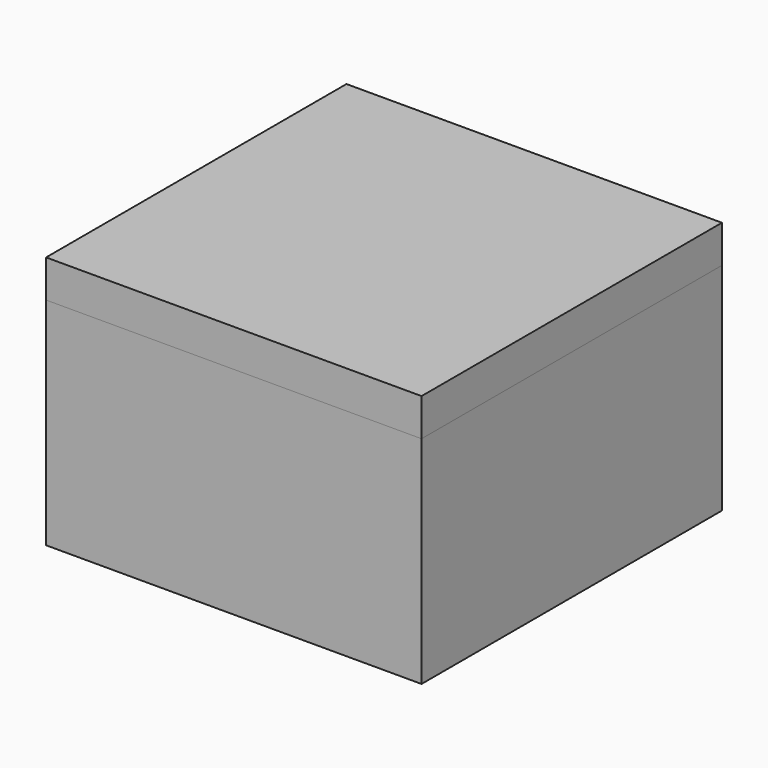
from build123d import *

# Parameters (mm, degrees)
F0_W     = 40
F0_H     = 40
F0_W_2   = 37
F0_H_2   = 37
F0_W_3   = 35
F0_H_3   = 35
F0_W_4   = 34
F0_H_4   = 34
F1_DEPTH = 2
F2_DEPTH = 25
F3_DEPTH = 23
F4_START = 23
F4_DEPTH = 4
F5_START = 25
F5_DEPTH = 2


with BuildPart() as f1:
    # F0 (on Top) → F1 (new body)
    with BuildSketch(Plane.XY):
        Rectangle(F0_W, F0_H)
        Rectangle(F0_W_2, F0_H_2, mode=Mode.SUBTRACT)
        Rectangle(F0_W_2, F0_H_2)
        Rectangle(F0_W_3, F0_H_3, mode=Mode.SUBTRACT)
        Rectangle(F0_W_3, F0_H_3)
        Rectangle(F0_W_4, F0_H_4, mode=Mode.SUBTRACT)
        Rectangle(F0_W_4, F0_H_4)
    extrude(amount=F1_DEPTH)

    # F0 (on Top) → F2 (join)
    with BuildSketch(Plane.XY):
        Rectangle(F0_W_2, F0_H_2)
        Rectangle(F0_W_3, F0_H_3, mode=Mode.SUBTRACT)
    extrude(amount=F2_DEPTH)

    # F0 (on Top) → F3 (join)
    with BuildSketch(Plane.XY):
        Rectangle(F0_W, F0_H)
        Rectangle(F0_W_2, F0_H_2, mode=Mode.SUBTRACT)
    extrude(amount=F3_DEPTH)


with BuildPart() as f4:
    # F0 (on Top) → F4 (new body)
    with BuildSketch(Plane.XY.offset(F4_START)):
        Rectangle(F0_W, F0_H)
        Rectangle(F0_W_2, F0_H_2, mode=Mode.SUBTRACT)
    extrude(amount=F4_DEPTH)

    # F0 (on Top) → F5 (join)
    with BuildSketch(Plane.XY.offset(F5_START)):
        Rectangle(F0_W_2, F0_H_2)
        Rectangle(F0_W_3, F0_H_3, mode=Mode.SUBTRACT)
        Rectangle(F0_W_3, F0_H_3)
        Rectangle(F0_W_4, F0_H_4, mode=Mode.SUBTRACT)
        Rectangle(F0_W_4, F0_H_4)
    extrude(amount=F5_DEPTH)


solid = Compound([f1.part, f4.part])
